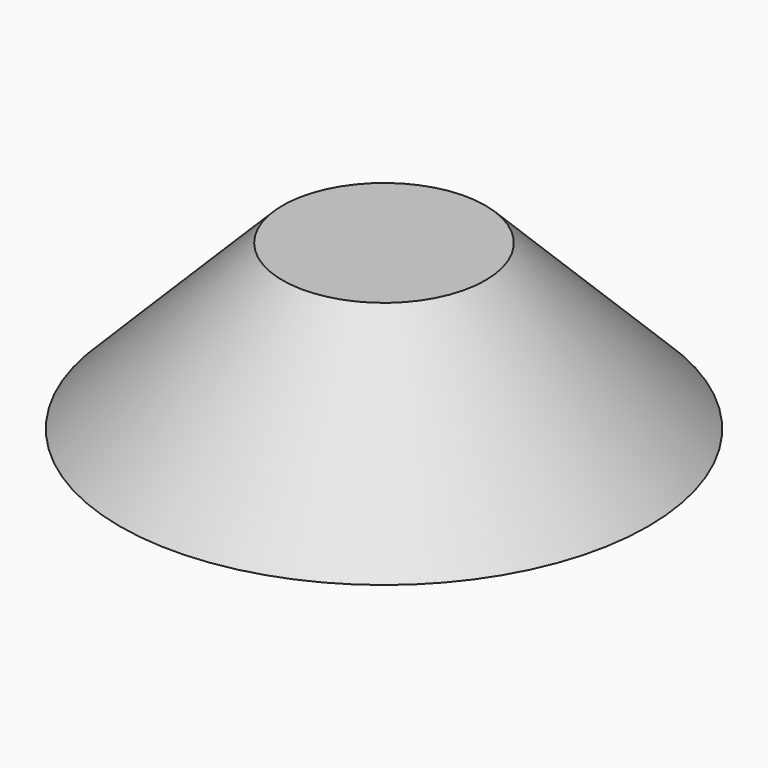
from build123d import *


# Not quite as in the source:
# - the program builds the solid bodies; features that only make, move or delete a surface that nothing else refers to are left out


with BuildPart() as f1:
    # F0 (on Front) → F1 (revolve)
    with BuildSketch(Plane.XZ):
        Polygon((-44.7060465813, 45.6278249621), (-63.3258894086, 45.6278249621), (-63.3258894086, 15.5779840425), (-14.8405646905, 15.5779840425), align=None)
    revolve(axis=Axis((-63.3258894086, 0, 30.6029045023), (0, 0, -1)))


solid = f1.part
